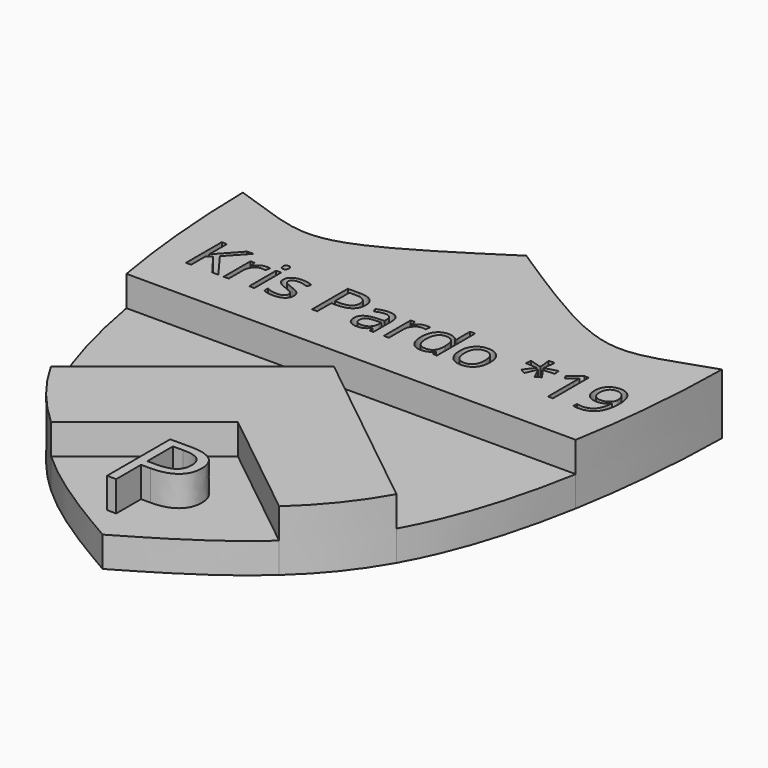
from build123d import *

# Parameters (mm, degrees)
F1_DEPTH     = 12.7
F2_DEPTH     = 12.7
F3_DEPTH     = 6.35
F4_DEPTH     = 6.35
F5_TEXT_SIZE = 13.1481524276
F6_DEPTH     = 6.35
F7_TEXT_SIZE = 23.1960429469
F8_DEPTH     = 6.35


# Not quite as in the source:
# - Text() gives the source's letters only with a copy of the font that has no kerning and outlines rounded to 1/6400 em; it was checked with that copy


with BuildPart() as f1:
    # F0 (on Top) → F1 (new body)
    with BuildSketch(Plane.XY):
        with BuildLine():
            Line((0, 5.4481513798), (-36.2691245973, -23.5048830509))
            add(Edge.make_bspline(
                [(-36.2691245973, -23.5048830509), (-32.8500376213, -29.5814165321), (-28.694092778, -34.537288094), (-23.9332160119, -38.8744926509)],
                knots=[0.5452445381, 0.5452445381, 0.5452445381, 0.5452445381, 0.7316320036, 0.7316320036, 0.7316320036, 0.7316320036], degree=3))
            Line((-23.9332160119, -38.8744926509), (0, -19.7690073401))
            Line((0, -19.7690073401), (23.9332160119, -38.8744926509))
            add(Edge.make_bspline(
                [(36.2691245973, -23.5048830509), (32.8500376213, -29.5814165321), (28.694092778, -34.537288094), (23.9332160119, -38.8744926509)],
                knots=[0.5452445381, 0.5452445381, 0.5452445381, 0.5452445381, 0.7316320036, 0.7316320036, 0.7316320036, 0.7316320036], degree=3))
            Line((36.2691245973, -23.5048830509), (0, 5.4481513798))
        make_face()
    extrude(amount=F1_DEPTH)



with BuildPart() as f2:
    # F0 (on Top) → F2 (new body)
    with BuildSketch(Plane.XY):
        with BuildLine():
            add(Edge.make_bspline(
                [(-50.27865991, 44.3635210395), (-41.0054572723, 41.1930002972), (-30.8844332128, 36.9428097603), (-17.55950923, 44.4225819381), (0, 55.8824725449)],
                knots=[0, 0, 0, 0, 0.421221742, 1, 1, 1, 1], degree=3))
            add(Edge.make_bspline(
                [(-50.27865991, 44.3635210395), (-50.1288617136, 33.4283674253), (-49.1953965933, 21.4191179011), (-47.1529008417, 9.9208939787)],
                knots=[0, 0, 0, 0, 0.262350676, 0.262350676, 0.262350676, 0.262350676], degree=3))
            Line((-47.1529008417, 9.9208939787), (47.1529008417, 9.9208939787))
            add(Edge.make_bspline(
                [(50.27865991, 44.3635210395), (50.1288617136, 33.4283674253), (49.1953965933, 21.4191179011), (47.1529008417, 9.9208939787)],
                knots=[0, 0, 0, 0, 0.262350676, 0.262350676, 0.262350676, 0.262350676], degree=3))
            add(Edge.make_bspline(
                [(50.27865991, 44.3635210395), (41.0054572723, 41.1930002972), (30.8844332128, 36.9428097603), (17.55950923, 44.4225819381), (0, 55.8824725449)],
                knots=[0, 0, 0, 0, 0.421221742, 1, 1, 1, 1], degree=3))
        make_face()
    extrude(amount=F2_DEPTH)


with BuildPart() as f1_1:
    add(f1.part)

    add(f2.part)  # F3 merges F2
    # F0 (on Top) → F3 (join)
    with BuildSketch(Plane.XY):
        with BuildLine():
            Line((47.1529008417, 9.9208939787), (-47.1529008417, 9.9208939787))
            add(Edge.make_bspline(
                [(-47.1529008417, 9.9208939787), (-44.9504688904, -2.4776903168), (-41.4585224822, -14.2820846207), (-36.2691245973, -23.5048830509)],
                knots=[0.262350676, 0.262350676, 0.262350676, 0.262350676, 0.5452445381, 0.5452445381, 0.5452445381, 0.5452445381], degree=3))
            Line((-36.2691245973, -23.5048830509), (0, 5.4481513798))
            Line((0, 5.4481513798), (36.2691245973, -23.5048830509))
            add(Edge.make_bspline(
                [(47.1529008417, 9.9208939787), (44.9504688904, -2.4776903168), (41.4585224822, -14.2820846207), (36.2691245973, -23.5048830509)],
                knots=[0.262350676, 0.262350676, 0.262350676, 0.262350676, 0.5452445381, 0.5452445381, 0.5452445381, 0.5452445381], degree=3))
        make_face()
        with BuildLine():
            Line((0, -19.7690073401), (-23.9332160119, -38.8744926509))
            add(Edge.make_bspline(
                [(-23.9332160119, -38.8744926509), (-17.0783185783, -45.1193701907), (-8.9693142797, -50.0816661556), (0, -55.2598275244)],
                knots=[0.7316320036, 0.7316320036, 0.7316320036, 0.7316320036, 1, 1, 1, 1], degree=3))
            add(Edge.make_bspline(
                [(23.9332160119, -38.8744926509), (17.0783185783, -45.1193701907), (8.9693142797, -50.0816661556), (0, -55.2598275244)],
                knots=[0.7316320036, 0.7316320036, 0.7316320036, 0.7316320036, 1, 1, 1, 1], degree=3))
            Line((23.9332160119, -38.8744926509), (0, -19.7690073401))
        make_face()
    extrude(amount=F3_DEPTH)

    # F0 (on Top) → F4 (join)
    with BuildSketch(Plane.XY):
        with BuildLine():
            add(Edge.make_bspline(
                [(-50.27865991, 44.3635210395), (-41.0054572723, 41.1930002972), (-30.8844332128, 36.9428097603), (-17.55950923, 44.4225819381), (0, 55.8824725449)],
                knots=[0, 0, 0, 0, 0.421221742, 1, 1, 1, 1], degree=3))
            add(Edge.make_bspline(
                [(-50.27865991, 44.3635210395), (-50.1288617136, 33.4283674253), (-49.1953965933, 21.4191179011), (-47.1529008417, 9.9208939787)],
                knots=[0, 0, 0, 0, 0.262350676, 0.262350676, 0.262350676, 0.262350676], degree=3))
            Line((-47.1529008417, 9.9208939787), (47.1529008417, 9.9208939787))
            add(Edge.make_bspline(
                [(50.27865991, 44.3635210395), (50.1288617136, 33.4283674253), (49.1953965933, 21.4191179011), (47.1529008417, 9.9208939787)],
                knots=[0, 0, 0, 0, 0.262350676, 0.262350676, 0.262350676, 0.262350676], degree=3))
            add(Edge.make_bspline(
                [(50.27865991, 44.3635210395), (41.0054572723, 41.1930002972), (30.8844332128, 36.9428097603), (17.55950923, 44.4225819381), (0, 55.8824725449)],
                knots=[0, 0, 0, 0, 0.421221742, 1, 1, 1, 1], degree=3))
        make_face()
        with BuildLine():
            Line((47.1529008417, 9.9208939787), (-47.1529008417, 9.9208939787))
            add(Edge.make_bspline(
                [(-47.1529008417, 9.9208939787), (-44.9504688904, -2.4776903168), (-41.4585224822, -14.2820846207), (-36.2691245973, -23.5048830509)],
                knots=[0.262350676, 0.262350676, 0.262350676, 0.262350676, 0.5452445381, 0.5452445381, 0.5452445381, 0.5452445381], degree=3))
            Line((-36.2691245973, -23.5048830509), (0, 5.4481513798))
            Line((0, 5.4481513798), (36.2691245973, -23.5048830509))
            add(Edge.make_bspline(
                [(47.1529008417, 9.9208939787), (44.9504688904, -2.4776903168), (41.4585224822, -14.2820846207), (36.2691245973, -23.5048830509)],
                knots=[0.262350676, 0.262350676, 0.262350676, 0.262350676, 0.5452445381, 0.5452445381, 0.5452445381, 0.5452445381], degree=3))
        make_face()
        with BuildLine():
            Line((0, 5.4481513798), (-36.2691245973, -23.5048830509))
            add(Edge.make_bspline(
                [(-36.2691245973, -23.5048830509), (-32.8500376213, -29.5814165321), (-28.694092778, -34.537288094), (-23.9332160119, -38.8744926509)],
                knots=[0.5452445381, 0.5452445381, 0.5452445381, 0.5452445381, 0.7316320036, 0.7316320036, 0.7316320036, 0.7316320036], degree=3))
            Line((-23.9332160119, -38.8744926509), (0, -19.7690073401))
            Line((0, -19.7690073401), (23.9332160119, -38.8744926509))
            add(Edge.make_bspline(
                [(36.2691245973, -23.5048830509), (32.8500376213, -29.5814165321), (28.694092778, -34.537288094), (23.9332160119, -38.8744926509)],
                knots=[0.5452445381, 0.5452445381, 0.5452445381, 0.5452445381, 0.7316320036, 0.7316320036, 0.7316320036, 0.7316320036], degree=3))
            Line((36.2691245973, -23.5048830509), (0, 5.4481513798))
        make_face()
        with BuildLine():
            Line((0, -19.7690073401), (-23.9332160119, -38.8744926509))
            add(Edge.make_bspline(
                [(-23.9332160119, -38.8744926509), (-17.0783185783, -45.1193701907), (-8.9693142797, -50.0816661556), (0, -55.2598275244)],
                knots=[0.7316320036, 0.7316320036, 0.7316320036, 0.7316320036, 1, 1, 1, 1], degree=3))
            add(Edge.make_bspline(
                [(23.9332160119, -38.8744926509), (17.0783185783, -45.1193701907), (8.9693142797, -50.0816661556), (0, -55.2598275244)],
                knots=[0.7316320036, 0.7316320036, 0.7316320036, 0.7316320036, 1, 1, 1, 1], degree=3))
            Line((23.9332160119, -38.8744926509), (0, -19.7690073401))
        make_face()
    extrude(amount=F4_DEPTH)

    # F5 (on face) → F6 (cut)
    with BuildSketch(Plane.XY.offset(12.7)):
        with Locations((-43.2626888585, 19.0714837904)):
            Text('Kris Pardo *19', F5_TEXT_SIZE, font='Open Sans', text_align=(TextAlign.LEFT, TextAlign.BOTTOM))
    extrude(amount=-F6_DEPTH, mode=Mode.SUBTRACT)

    # F7 (on face) → F8 (join)
    with BuildSketch(Plane.XY.offset(6.35)):
        with Locations((-7.1400319696, -48.0265023687)):
            Text('P', F7_TEXT_SIZE, font='Open Sans', text_align=(TextAlign.LEFT, TextAlign.BOTTOM))
    extrude(amount=F8_DEPTH)


solid = f1_1.part
